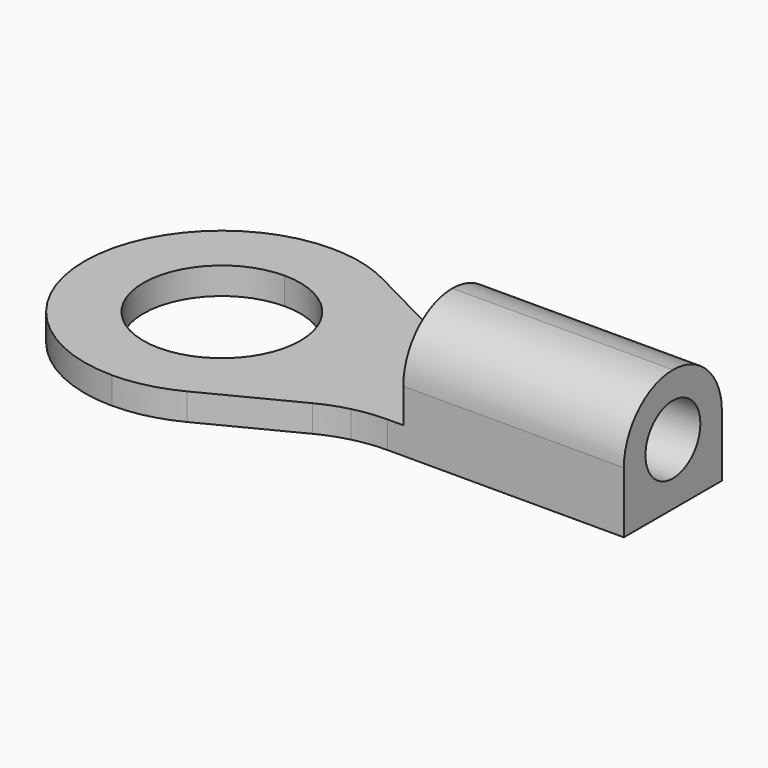
from build123d import *

# Parameters (mm, degrees)
F1_DEPTH = 0.55
F2_W     = 4.5
F2_H     = 2.5
F3_DEPTH = 1.95
F4_R     = 1.24999
F5_R     = 0.7
F6_DEPTH = 25


# Not quite as in the source:
# - a fillet or chamfer is up to 0.001 mm smaller than in the source, because OpenCascade refuses the exact size


with BuildPart() as f1:
    # F0 (on Top) → F1 (new body)
    with BuildSketch(Plane.XY):
        with BuildLine():
            Line((7.1757397782, 1.55), (12, 1.55))
            Line((12, 1.55), (12, 4.05))
            Line((12, 4.05), (7.1757397782, 4.05))
            ThreePointArc((7.1757397782, 4.05), (6.8353451552, 4.0707678217), (6.5, 4.1327632138))
            ThreePointArc((6.5, 4.1327632138), (6.1928359056, 4.2281876541), (5.8986420809, 4.3582091838))
            Line((5.8986420809, 4.3582091838), (4.0770976972, 5.2917908162))
            ThreePointArc((4.0770976972, 5.2917908162), (3.4568811592, 5.5218572965), (2.8, 5.6))
            Line((2.8, 5.6), (2.8, 4.4))
            ThreePointArc((2.8, 4.4), (3.9313708499, 3.9313708499), (4.4, 2.8))
            ThreePointArc((4.4, 2.8), (3.9313708499, 1.6686291501), (2.8, 1.2))
            Line((2.8, 1.2), (2.8, 0))
            ThreePointArc((2.8, 0), (3.4568811592, 0.0781427035), (4.0770976972, 0.3082091838))
            Line((4.0770976972, 0.3082091838), (5.8986420809, 1.2417908162))
            ThreePointArc((5.8986420809, 1.2417908162), (6.1928359056, 1.3718123459), (6.5, 1.4672367862))
            ThreePointArc((6.5, 1.4672367862), (6.8353451552, 1.5292321783), (7.1757397782, 1.55))
        make_face()
        with BuildLine():
            ThreePointArc((0, 2.8), (0.8201010127, 0.8201010127), (2.8, 0))
            Line((2.8, 0), (2.8, 1.2))
            ThreePointArc((2.8, 1.2), (1.2, 2.8), (2.8, 4.4))
            Line((2.8, 4.4), (2.8, 5.6))
            ThreePointArc((2.8, 5.6), (0.8201010127, 4.7798989873), (0, 2.8))
        make_face()
    extrude(amount=F1_DEPTH)

    # F2 (on face) → F3 (join)
    with BuildSketch(Plane.XY.offset(0.55)):
        with Locations((9.75, 2.8)):
            Rectangle(F2_W, F2_H)
    extrude(amount=F3_DEPTH)

    # F4 (radius 1.25 in the source; OpenCascade refuses exactly that, so slightly less here)
    f4_edges = [f1.edges().sort_by_distance(p)[0] for p in [
        (9.75, 1.55, 2.5),
        (9.75, 4.05, 2.5),
    ]]
    fillet(f4_edges, radius=F4_R)

    # F5 (on face) → F6 (cut)
    with BuildSketch(Plane.YZ.offset(12)):
        with Locations((2.8, 1.25)):
            Circle(F5_R)
    extrude(amount=-F6_DEPTH, mode=Mode.SUBTRACT)


solid = f1.part
